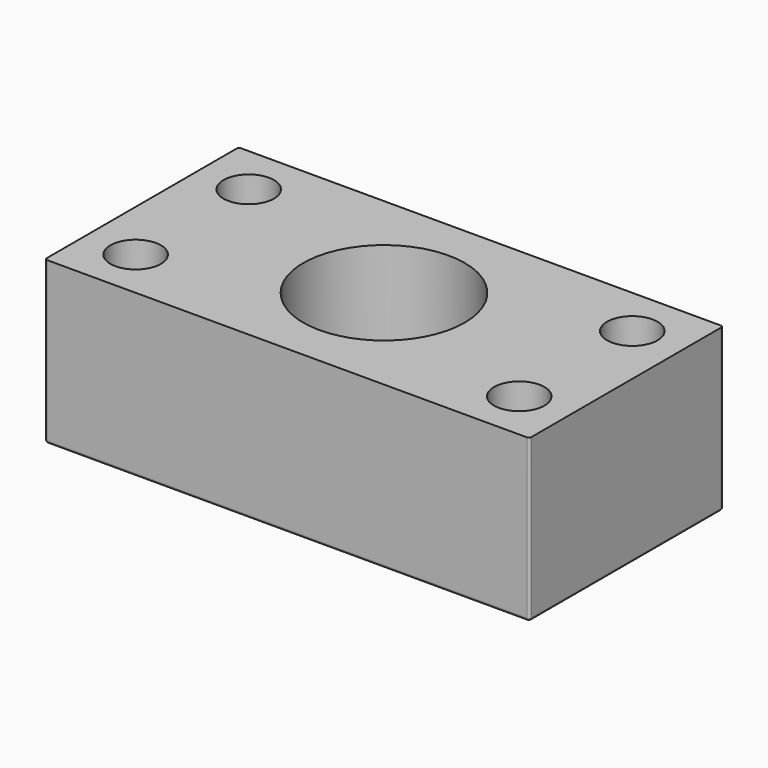
from build123d import *

# Parameters (mm, degrees)
F0_W         = 76.2
F0_H         = 38.1
F0_R         = 3.96875
F1_DEPTH     = 25.4
F2_R         = 0.381
F3_R         = 0.381
F4_T1_DEPTH  = 25.9715
F4_S5_W      = 0.381
F4_S5_H      = 0.381
F4_T6_DEPTH  = 0.381
F4_S11_W     = 0.381
F4_S11_H     = 0.381
F4_T12_DEPTH = 0.381
F5_R         = 12.7
F6_DEPTH     = 25.4
F7_R         = 15.875
F8_DEPTH     = 4.7625
F9_SIZE      = 0.381


# Not quite as in the source:
# - a fillet or chamfer that OpenCascade refuses, or shapes differently, is made with other operations: its cross-section is extruded or revolved along the edge and cut away or added


with BuildPart() as f1:
    # F0 (on Top) → F1 (new body)
    with BuildSketch(Plane.XY):
        Rectangle(F0_W, F0_H)
        with Locations((-30.1625, -11.1125)):
            Circle(F0_R, mode=Mode.SUBTRACT)
        with Locations((30.1625, -11.1125)):
            Circle(F0_R, mode=Mode.SUBTRACT)
        with Locations((-30.1625, 11.1125)):
            Circle(F0_R, mode=Mode.SUBTRACT)
        with Locations((30.1625, 11.1125)):
            Circle(F0_R, mode=Mode.SUBTRACT)
    extrude(amount=F1_DEPTH)

    # F2
    f2_edges = [f1.edges().sort_by_distance(p)[0] for p in [
        (0, -19.05, 0),
        (38.1, 0, 0),
        (-38.1, 0, 0),
    ]]
    fillet(f2_edges, radius=F2_R)

    # F3
    f3_edges = [f1.edges().sort_by_distance(p)[0] for p in [
        (0, 19.05, 0),
    ]]
    fillet(f3_edges, radius=F3_R)

    # F4: fillet of radius 0.381 on 3 edges, made by hand

    # F4_s2 → F4_t1 (cut)
    with BuildSketch(Plane.XY.offset(0.381)):
        with BuildLine():
            ThreePointArc((38.1, -18.669), (37.9884076836, -18.9384076836), (37.719, -19.05))
            Line((37.719, -19.05), (38.1, -19.05))
            Line((38.1, -19.05), (38.1, -18.669))
        make_face()
        with BuildLine():
            ThreePointArc((-37.719, -19.05), (-37.9884076836, -18.9384076836), (-38.1, -18.669))
            Line((-38.1, -18.669), (-38.1, -19.05))
            Line((-38.1, -19.05), (-37.719, -19.05))
        make_face()
    extrude(amount=F4_T1_DEPTH, mode=Mode.SUBTRACT)


with BuildPart() as f4_tool4:
    # F4_s5 → F4_t6 (new body)
    with BuildSketch(Plane.XZ.offset(18.669)):
        with Locations((-37.9095, 0.1905)):
            Rectangle(F4_S5_W, F4_S5_H)
    extrude(amount=F4_T6_DEPTH)

    # F4_s7 → F4_t8 (revolve, cut)
    with BuildSketch(Plane(origin=(-37.719, -18.669, 0.381), x_dir=(0.7071067812, 0, 0.7071067812), z_dir=(0.7071067812, 0, -0.7071067812))):
        with BuildLine():
            ThreePointArc((0, -0.381), (0.381, 0), (0, 0.381))
            Line((0, 0.381), (0, -0.381))
        make_face()
    revolve(axis=Axis((-37.719, -18.669, 0.381), (0, -1, 0)), mode=Mode.SUBTRACT)


with BuildPart() as f1_1:
    add(f1.part)

    # F4_t3: cut F4_tool4
    add(f4_tool4.part, mode=Mode.SUBTRACT)


with BuildPart() as f4_tool10:
    # F4_s11 → F4_t12 (new body)
    with BuildSketch(Plane.YZ.offset(37.719)):
        with Locations((-18.8595, 0.1905)):
            Rectangle(F4_S11_W, F4_S11_H)
    extrude(amount=F4_T12_DEPTH)

    # F4_s13 → F4_t14 (revolve, cut)
    with BuildSketch(Plane(origin=(37.719, -18.669, 0.381), x_dir=(0, 0.7071067812, 0.7071067812), z_dir=(0, 0.7071067812, -0.7071067812))):
        with BuildLine():
            ThreePointArc((0, -0.381), (0.381, 0), (0, 0.381))
            Line((0, 0.381), (0, -0.381))
        make_face()
    revolve(axis=Axis((37.719, -18.669, 0.381), (1, 0, 0)), mode=Mode.SUBTRACT)


with BuildPart() as f1_2:
    add(f1_1.part)

    # F4_t9: cut F4_tool10
    add(f4_tool10.part, mode=Mode.SUBTRACT)

    # F5 (on face) → F6 (cut)
    with BuildSketch(Plane.XY.offset(25.4)):
        Circle(F5_R)
    extrude(amount=-F6_DEPTH, mode=Mode.SUBTRACT)

    # F7 (on face) → F8 (cut)
    with BuildSketch(Plane(origin=(0, 0, 0), x_dir=(1, 0, 0), z_dir=(0, 0, -1))):
        Circle(F7_R)
    extrude(amount=-F8_DEPTH, mode=Mode.SUBTRACT)

    # F9
    f9_edges = [f1_2.edges().sort_by_distance(p)[0] for p in [
        (-12.7, 0, 4.7625),
    ]]
    chamfer(f9_edges, length=F9_SIZE)


solid = f1_2.part
